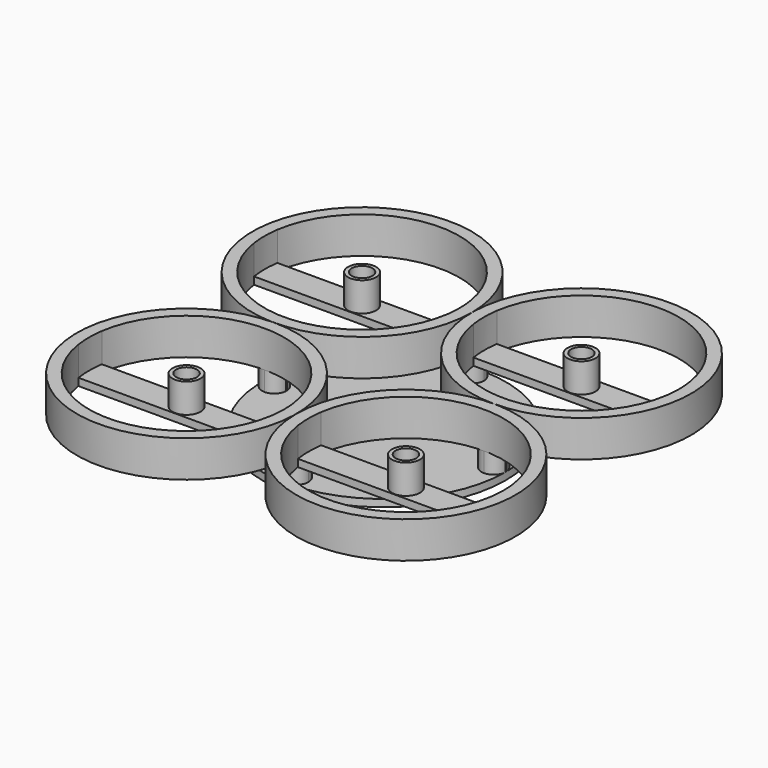
from build123d import *

# Parameters (mm, degrees)
F1_DEPTH = 15
F0_R     = 5.75
F2_DEPTH = 3
F0_R_2   = 4.25
F3_DEPTH = 15
F5_DEPTH = 8
F6_R     = 50
F7_DEPTH = 3


# Not quite as in the source:
# - a feature names something its author has since deleted; it is built from what else it names


with BuildPart() as f1:
    # F0 (on Top) → F1 (new body)
    with BuildSketch(Plane.XY):
        with BuildLine():
            ThreePointArc((-45, 0), (-13.1801948466, 13.1801948466), (0, 45))
            ThreePointArc((0, 45), (-76.8198051534, 76.8198051534), (-45, 0))
        make_face()
        with BuildLine():
            ThreePointArc((-5.4525601334, 51), (-5.1133004959, 48.0085216749), (-5, 45))
            ThreePointArc((-5, 45), (-5.1133004959, 41.9914783251), (-5.4525601334, 39))
            ThreePointArc((-5.4525601334, 39), (-45, 5), (-84.5474398666, 39))
            ThreePointArc((-84.5474398666, 39), (-85, 45), (-84.5474398666, 51))
            ThreePointArc((-84.5474398666, 51), (-45, 85), (-5.4525601334, 51))
        make_face(mode=Mode.SUBTRACT)
    extrude(amount=F1_DEPTH)


with BuildPart() as f1b:
    # F0 (on Top) → F1, piece 2 (new body)
    with BuildSketch(Plane.XY):
        with BuildLine():
            ThreePointArc((90, 45), (45, 90), (0, 45))
            ThreePointArc((0, 45), (13.1801949066, 13.1801947866), (45.0000001696, 0))
            ThreePointArc((45.0000001696, 0), (76.8198052134, 13.1801949066), (90, 45))
        make_face()
        with BuildLine():
            ThreePointArc((84.5474398666, 51), (84.8866995041, 48.0085216749), (85, 45))
            ThreePointArc((85, 45), (84.8866995041, 41.9914783251), (84.5474398666, 39))
            ThreePointArc((84.5474398666, 39), (45, 5), (5.4525601334, 39))
            ThreePointArc((5.4525601334, 39), (5, 45), (5.4525601334, 51))
            ThreePointArc((5.4525601334, 51), (45, 85), (84.5474398666, 51))
        make_face(mode=Mode.SUBTRACT)
    extrude(amount=F1_DEPTH)


with BuildPart() as f1c:
    # F0 (on Top) → F1, piece 3 (new body)
    with BuildSketch(Plane.XY):
        with BuildLine():
            ThreePointArc((0, -45), (-13.1801948466, -13.1801948466), (-45, 0))
            ThreePointArc((-45, 0), (-76.8198051534, -76.8198051534), (0, -45))
        make_face()
        with BuildLine():
            ThreePointArc((-5.4525601334, -39), (-5.1133004959, -41.9914783251), (-5, -45))
            ThreePointArc((-5, -45), (-5.1133004959, -48.0085216749), (-5.4525601334, -51))
            ThreePointArc((-5.4525601334, -51), (-45, -85), (-84.5474398666, -51))
            ThreePointArc((-84.5474398666, -51), (-85, -45), (-84.5474398666, -39))
            ThreePointArc((-84.5474398666, -39), (-45, -5), (-5.4525601334, -39))
        make_face(mode=Mode.SUBTRACT)
    extrude(amount=F1_DEPTH)


with BuildPart() as f1d:
    # F0 (on Top) → F1, piece 4 (new body)
    with BuildSketch(Plane.XY):
        with BuildLine():
            ThreePointArc((90, -45), (76.8198052134, -13.1801949066), (45.0000001696, 0))
            ThreePointArc((45.0000001696, 0), (13.1801949066, -13.1801947866), (0, -45))
            ThreePointArc((0, -45), (45, -90), (90, -45))
        make_face()
        with BuildLine():
            ThreePointArc((84.5474398666, -39), (84.8866995041, -41.9914783251), (85, -45))
            ThreePointArc((85, -45), (84.8866995041, -48.0085216749), (84.5474398666, -51))
            ThreePointArc((84.5474398666, -51), (45, -85), (5.4525601334, -51))
            ThreePointArc((5.4525601334, -51), (5, -45), (5.4525601334, -39))
            ThreePointArc((5.4525601334, -39), (45, -5), (84.5474398666, -39))
        make_face(mode=Mode.SUBTRACT)
    extrude(amount=F1_DEPTH)


with BuildPart() as f2:
    # F0 (on Top) → F2 (new body)
    with BuildSketch(Plane.XY):
        with BuildLine():
            ThreePointArc((84.5474398666, -51), (84.8866995041, -48.0085216749), (85, -45))
            ThreePointArc((85, -45), (84.8866995041, -41.9914783251), (84.5474398666, -39))
            Line((84.5474398666, -39), (5.4525601334, -39))
            ThreePointArc((5.4525601334, -39), (5, -45), (5.4525601334, -51))
            Line((5.4525601334, -51), (84.5474398666, -51))
        make_face()
        with Locations((45, -45)):
            Circle(F0_R, mode=Mode.SUBTRACT)
    extrude(amount=F2_DEPTH)


with BuildPart() as f2b:
    # F0 (on Top) → F2, piece 2 (new body)
    with BuildSketch(Plane.XY):
        with BuildLine():
            ThreePointArc((84.5474398666, 39), (84.8866995041, 41.9914783251), (85, 45))
            ThreePointArc((85, 45), (84.8866995041, 48.0085216749), (84.5474398666, 51))
            Line((84.5474398666, 51), (5.4525601334, 51))
            ThreePointArc((5.4525601334, 51), (5, 45), (5.4525601334, 39))
            Line((5.4525601334, 39), (84.5474398666, 39))
        make_face()
        with Locations((45, 45)):
            Circle(F0_R, mode=Mode.SUBTRACT)
    extrude(amount=F2_DEPTH)


with BuildPart() as f2c:
    # F0 (on Top) → F2, piece 3 (new body)
    with BuildSketch(Plane.XY):
        with BuildLine():
            ThreePointArc((-5.4525601334, 39), (-5.1133004959, 41.9914783251), (-5, 45))
            ThreePointArc((-5, 45), (-5.1133004959, 48.0085216749), (-5.4525601334, 51))
            Line((-5.4525601334, 51), (-84.5474398666, 51))
            ThreePointArc((-84.5474398666, 51), (-85, 45), (-84.5474398666, 39))
            Line((-84.5474398666, 39), (-5.4525601334, 39))
        make_face()
        with Locations((-45, 45)):
            Circle(F0_R, mode=Mode.SUBTRACT)
    extrude(amount=F2_DEPTH)


with BuildPart() as f2d:
    # F0 (on Top) → F2, piece 4 (new body)
    with BuildSketch(Plane.XY):
        with BuildLine():
            ThreePointArc((-5.4525601334, -51), (-5.1133004959, -48.0085216749), (-5, -45))
            ThreePointArc((-5, -45), (-5.1133004959, -41.9914783251), (-5.4525601334, -39))
            Line((-5.4525601334, -39), (-84.5474398666, -39))
            ThreePointArc((-84.5474398666, -39), (-85, -45), (-84.5474398666, -51))
            Line((-84.5474398666, -51), (-5.4525601334, -51))
        make_face()
        with Locations((-45, -45)):
            Circle(F0_R, mode=Mode.SUBTRACT)
    extrude(amount=F2_DEPTH)


with BuildPart() as f3:
    # F0 (on Top) → F3 (new body)
    with BuildSketch(Plane.XY):
        with Locations((-45, 45)):
            Circle(F0_R)
        with Locations((-45, 45)):
            Circle(F0_R_2, mode=Mode.SUBTRACT)
    extrude(amount=F3_DEPTH)


with BuildPart() as f3b:
    # F0 (on Top) → F3, piece 2 (new body)
    with BuildSketch(Plane.XY):
        with Locations((45, 45)):
            Circle(F0_R)
        with Locations((45, 45)):
            Circle(F0_R_2, mode=Mode.SUBTRACT)
    extrude(amount=F3_DEPTH)


with BuildPart() as f3c:
    # F0 (on Top) → F3, piece 3 (new body)
    with BuildSketch(Plane.XY):
        with Locations((-45, -45)):
            Circle(F0_R)
        with Locations((-45, -45)):
            Circle(F0_R_2, mode=Mode.SUBTRACT)
    extrude(amount=F3_DEPTH)


with BuildPart() as f3d:
    # F0 (on Top) → F3, piece 4 (new body)
    with BuildSketch(Plane.XY):
        with Locations((45, -45)):
            Circle(F0_R)
        with Locations((45, -45)):
            Circle(F0_R_2, mode=Mode.SUBTRACT)
    extrude(amount=F3_DEPTH)


with BuildPart() as f5:
    # F4 (on Top) → F5 (new body)
    with BuildSketch(Plane.XY):
        with BuildLine():
            ThreePointArc((-0.2777777778, -49.9922779877), (-0.069498111, -47.5), (0, -45))
            ThreePointArc((0, -45), (-0.069498111, -42.5), (-0.2777777778, -40.0077220123))
            ThreePointArc((-0.2777777778, -40.0077220123), (-3.6324157863, -41.5640786453), (-5, -45))
            ThreePointArc((-5, -45), (-3.6324157863, -48.4359213547), (-0.2777777778, -49.9922779877))
        make_face()
    extrude(amount=-F5_DEPTH)


with BuildPart() as f5b:
    # F4 (on Top) → F5, piece 2 (new body)
    with BuildSketch(Plane.XY):
        with BuildLine():
            ThreePointArc((0.2777777778, -40.0077220123), (0.069498111, -42.5), (0, -45))
            ThreePointArc((0, -45), (0.069498111, -47.5), (0.2777777778, -49.9922779877))
            ThreePointArc((0.2777777778, -49.9922779877), (3.6324157863, -48.4359213547), (5, -45))
            ThreePointArc((5, -45), (3.6324157863, -41.5640786453), (0.2777777778, -40.0077220123))
        make_face()
    extrude(amount=-F5_DEPTH)


with BuildPart() as f5c:
    # F4 (on Top) → F5, piece 3 (new body)
    with BuildSketch(Plane.XY):
        with BuildLine():
            ThreePointArc((-45, -5), (-41.5640786453, -3.6324157863), (-40.0077220123, -0.2777777778))
            ThreePointArc((-40.0077220123, -0.2777777778), (-42.4999999989, -0.069498111), (-44.9999999978, 0))
            ThreePointArc((-44.9999999978, 0), (-47.4999999989, -0.0694981109), (-49.9922779877, -0.2777777778))
            ThreePointArc((-49.9922779877, -0.2777777778), (-48.4359213547, -3.6324157863), (-45, -5))
        make_face()
    extrude(amount=-F5_DEPTH)


with BuildPart() as f5d:
    # F4 (on Top) → F5, piece 4 (new body)
    with BuildSketch(Plane.XY):
        with BuildLine():
            ThreePointArc((45.0000000896, 0), (42.5000000447, -0.0694981085), (40.0077220123, -0.2777777778))
            ThreePointArc((40.0077220123, -0.2777777778), (41.5640786453, -3.6324157863), (45, -5))
            ThreePointArc((45, -5), (48.4359213547, -3.6324157863), (49.9922779877, -0.2777777778))
            ThreePointArc((49.9922779877, -0.2777777778), (47.5000000447, -0.0694981135), (45.0000000896, 0))
        make_face()
    extrude(amount=-F5_DEPTH)


with BuildPart() as f5e:
    # F4 (on Top) → F5, piece 5 (new body)
    with BuildSketch(Plane.XY):
        with BuildLine():
            ThreePointArc((-49.9922779877, 0.2777777778), (-47.4999999989, 0.0694981109), (-44.9999999978, 0))
            ThreePointArc((-44.9999999978, 0), (-42.4999999989, 0.069498111), (-40.0077220123, 0.2777777778))
            ThreePointArc((-40.0077220123, 0.2777777778), (-41.5640786453, 3.6324157863), (-45, 5))
            ThreePointArc((-45, 5), (-48.4359213547, 3.6324157863), (-49.9922779877, 0.2777777778))
        make_face()
    extrude(amount=-F5_DEPTH)


with BuildPart() as f5f:
    # F4 (on Top) → F5, piece 6 (new body)
    with BuildSketch(Plane.XY):
        with BuildLine():
            ThreePointArc((40.0077220123, 0.2777777778), (42.5000000447, 0.0694981085), (45.0000000896, 0))
            ThreePointArc((45.0000000896, 0), (47.5000000447, 0.0694981135), (49.9922779877, 0.2777777778))
            ThreePointArc((49.9922779877, 0.2777777778), (48.4359214017, 3.6324157418), (45.0000001294, 5))
            ThreePointArc((45.0000001294, 5), (41.5640786923, 3.6324158307), (40.0077220123, 0.2777777778))
        make_face()
    extrude(amount=-F5_DEPTH)


with BuildPart() as f5g:
    # F4 (on Top) → F5, piece 7 (new body)
    with BuildSketch(Plane.XY):
        with BuildLine():
            ThreePointArc((0, 45), (-0.069498111, 47.5), (-0.2777777778, 49.9922779877))
            ThreePointArc((-0.2777777778, 49.9922779877), (-3.6324157863, 48.4359213547), (-5, 45))
            ThreePointArc((-5, 45), (-3.6324157863, 41.5640786453), (-0.2777777778, 40.0077220123))
            ThreePointArc((-0.2777777778, 40.0077220123), (-0.069498111, 42.5), (0, 45))
        make_face()
    extrude(amount=-F5_DEPTH)


with BuildPart() as f5h:
    # F4 (on Top) → F5, piece 8 (new body)
    with BuildSketch(Plane.XY):
        with BuildLine():
            ThreePointArc((0, 45), (0.069498111, 42.5), (0.2777777778, 40.0077220123))
            ThreePointArc((0.2777777778, 40.0077220123), (3.6324157863, 41.5640786453), (5, 45))
            ThreePointArc((5, 45), (3.6324157863, 48.4359213547), (0.2777777778, 49.9922779877))
            ThreePointArc((0.2777777778, 49.9922779877), (0.069498111, 47.5), (0, 45))
        make_face()
    extrude(amount=-F5_DEPTH)


with BuildPart() as f7:
    # F6 (on face) → F7 (new body)
    with BuildSketch(Plane(origin=(0, 0, -8), x_dir=(1, 0, 0), z_dir=(0, 0, -1))):
        Circle(F6_R)
        with BuildLine():
            ThreePointArc((-40.0077220123, -0.2777777778), (-45, -5), (-49.9922779877, -0.2777777778))
            ThreePointArc((-49.9922779877, -0.2777777778), (-45, 0), (-40.0077220123, -0.2777777778))
        make_face(mode=Mode.SUBTRACT)
        with BuildLine():
            ThreePointArc((-40.0077220123, -0.2777777778), (-45, 0), (-49.9922779877, -0.2777777778))
            ThreePointArc((-49.9922779877, -0.2777777778), (-45, -5), (-40.0077220123, -0.2777777778))
        make_face()
    extrude(amount=F7_DEPTH)


solid = Compound([f1.part, f1b.part, f1c.part, f1d.part, f2.part, f2b.part, f2c.part, f2d.part, f3.part, f3b.part, f3c.part, f3d.part, f5.part, f5b.part, f5c.part, f5d.part, f5e.part, f5f.part, f5g.part, f5h.part, f7.part])
